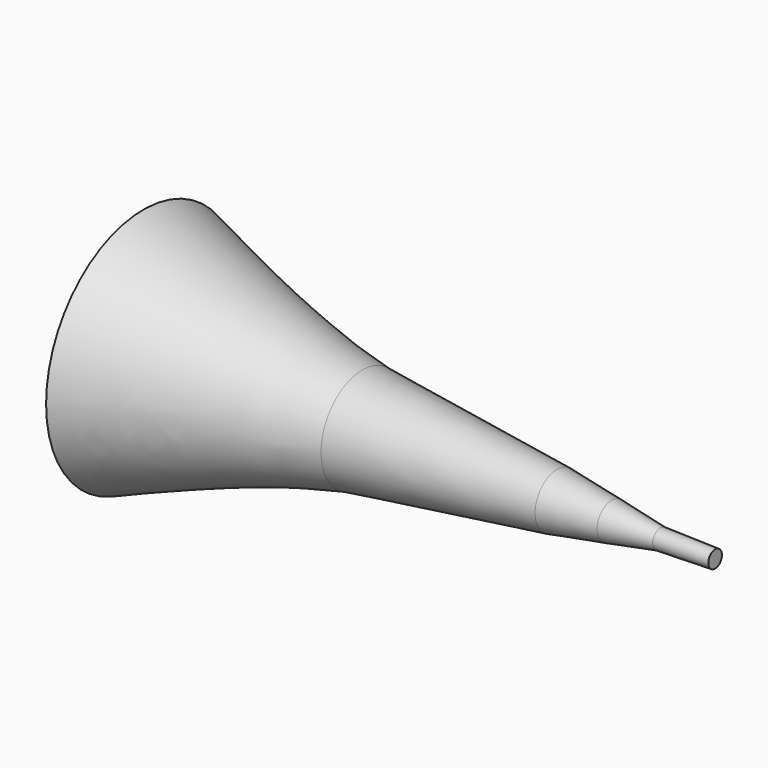
from build123d import *


with BuildPart() as f1:
    # F0 (on Top) → F1 (revolve)
    with BuildSketch(Plane.XY):
        with BuildLine():
            add(Edge.make_bspline(
                [(0, 0), (-38.4107541448, -6.923547728), (-76.8215082895, -13.847095456), (-114.3, -20.32)],
                knots=[0, 0, 0, 0, 0.145916612, 0.145916612, 0.145916612, 0.145916612], degree=3))
            Line((0, 0), (-114.3, 0))
            Line((-114.3, 0), (-114.3, -20.32))
        make_face()
        with BuildLine():
            Line((0, -17.78), (0, 0))
            add(Edge.make_bspline(
                [(0, 0), (-38.4107541448, -6.923547728), (-76.8215082895, -13.847095456), (-114.3, -20.32)],
                knots=[0, 0, 0, 0, 0.145916612, 0.145916612, 0.145916612, 0.145916612], degree=3))
            Line((-114.3, -20.32), (0, -17.78))
        make_face()
        with BuildLine():
            Line((-114.3, -20.32), (-114.3, 0))
            Line((-114.3, 0), (-215.9, 0))
            Line((-215.9, 0), (-215.9, -38.1))
            add(Edge.make_bspline(
                [(-114.3, -20.32), (-149.6266665218, -26.4212631464), (-184.1250490049, -32.1221448737), (-215.9, -38.1)],
                knots=[0.145916612, 0.145916612, 0.145916612, 0.145916612, 0.2834554311, 0.2834554311, 0.2834554311, 0.2834554311], degree=3))
        make_face()
        with BuildLine():
            Line((-215.9, -38.1), (-114.3, -20.32))
            add(Edge.make_bspline(
                [(-114.3, -20.32), (-149.6266665218, -26.4212631464), (-184.1250490049, -32.1221448737), (-215.9, -38.1)],
                knots=[0.145916612, 0.145916612, 0.145916612, 0.145916612, 0.2834554311, 0.2834554311, 0.2834554311, 0.2834554311], degree=3))
        make_face()
        Polygon((-215.9, -38.1), (-215.9, 0), (-330.2, 0), (-330.2, -57.15), align=None)
        with BuildLine():
            Line((-330.2, -57.15), (-330.2, 0))
            Line((-330.2, 0), (-736.6, 0))
            Line((-736.6, 0), (-736.6, -107.95))
            add(Edge.make_bspline(
                [(-330.2, -57.15), (-424.2035468422, -68.5554317066), (-586.7118007059, -77.9087616289), (-736.6, -107.95)],
                knots=[0.4292365201, 0.4292365201, 0.4292365201, 0.4292365201, 0.7033077599, 0.7033077599, 0.7033077599, 0.7033077599], degree=3))
        make_face()
        with BuildLine():
            Line((-736.6, -107.95), (-330.2, -57.15))
            add(Edge.make_bspline(
                [(-330.2, -57.15), (-424.2035468422, -68.5554317066), (-586.7118007059, -77.9087616289), (-736.6, -107.95)],
                knots=[0.4292365201, 0.4292365201, 0.4292365201, 0.4292365201, 0.7033077599, 0.7033077599, 0.7033077599, 0.7033077599], degree=3))
        make_face()
        with BuildLine():
            Line((-736.6, -107.95), (-736.6, 0))
            Line((-736.6, 0), (-1193.8, 0))
            Line((-1193.8, 0), (-1193.8, -254))
            add(Edge.make_bspline(
                [(-736.6, -107.95), (-898.8595120127, -140.4707501412), (-1046.3297560064, -197.2353750706), (-1193.8, -254)],
                knots=[0.7033077599, 0.7033077599, 0.7033077599, 0.7033077599, 1, 1, 1, 1], degree=3))
        make_face()
    revolve(axis=Axis((-965.2, 0, 0), (-1, 0, 0)))


solid = f1.part
